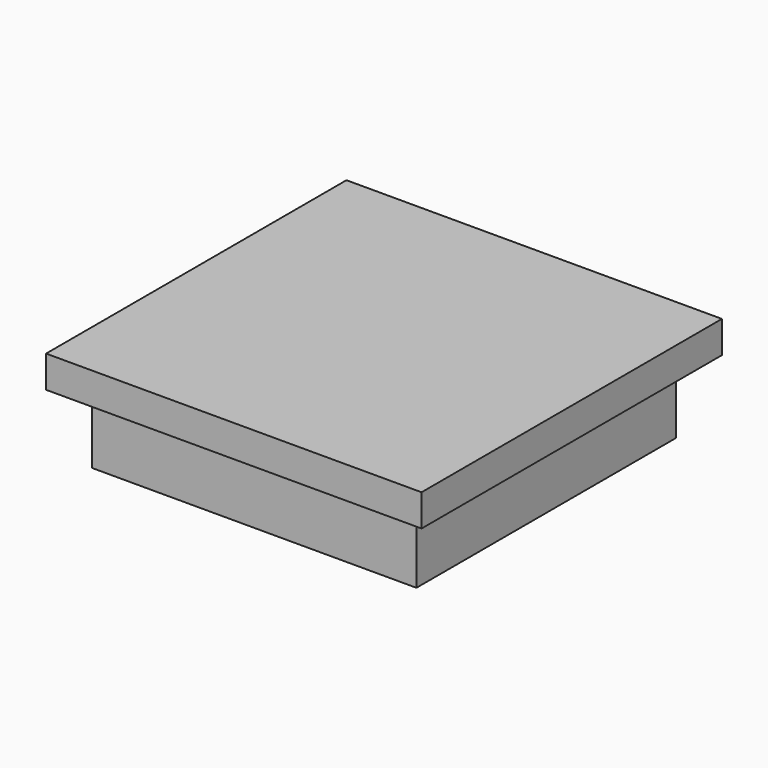
from build123d import *

# Parameters (mm, degrees)
F0_W     = 50.8
F0_H     = 50.8
F0_W_2   = 1
F0_H_2   = 8.95
F0_H_3   = 3
F1_DEPTH = 15
F2_DEPTH = 2
F3_R     = 5
F5_W     = 58.8
F5_H     = 58.8
F5_W_2   = 54.8
F5_H_2   = 54.8
F6_DEPTH = 5
F5_W_3   = 50.8
F5_H_3   = 50.8
F7_DEPTH = 2


with BuildPart() as f1:
    # F0 (on Top) → F1 (new body)
    with BuildSketch(Plane.XY):
        with Locations((-5.4668284297, -0.6229165018)):
            Rectangle(F0_W, F0_H)
        Polygon((-27.8668284297, 12.8270834982), (-27.8668284297, 21.7770834982), (-6.4668284297, 21.7770834982), (-5.4668284297, 21.7770834982), (-4.4668284297, 21.7770834982), (16.9331715703, 21.7770834982), (16.9331715703, 12.8270834982), (16.9331715703, 9.8270834982), (16.9331715703, 0.8770834982), (16.9331715703, -2.1229165018), (16.9331715703, -11.0729165018), (16.9331715703, -14.0729165018), (16.9331715703, -23.0229165018), (-4.4668284297, -23.0229165018), (-5.4668284297, -23.0229165018), (-6.4668284297, -23.0229165018), (-27.8668284297, -23.0229165018), (-27.8668284297, -14.0729165018), (-27.8668284297, -11.0729165018), (-27.8668284297, -2.1229165018), (-27.8668284297, 0.8770834982), (-27.8668284297, 9.8270834982), align=None, mode=Mode.SUBTRACT)
        with Locations((-5.9668284297, -6.5979165018)):
            Rectangle(F0_W_2, F0_H_2)
        with Locations((-4.9668284297, -6.5979165018)):
            Rectangle(F0_W_2, F0_H_2)
        with Locations((-5.9668284297, -12.5729165018)):
            Rectangle(F0_W_2, F0_H_3)
        with Locations((-4.9668284297, -12.5729165018)):
            Rectangle(F0_W_2, F0_H_3)
        with Locations((-5.9668284297, -18.5479165018)):
            Rectangle(F0_W_2, F0_H_2)
        with Locations((-4.9668284297, -18.5479165018)):
            Rectangle(F0_W_2, F0_H_2)
        with Locations((-5.9668284297, -0.6229165018)):
            Rectangle(F0_W_2, F0_H_3)
        with Locations((-4.9668284297, -0.6229165018)):
            Rectangle(F0_W_2, F0_H_3)
        with Locations((-5.9668284297, 5.3520834982)):
            Rectangle(F0_W_2, F0_H_2)
        with Locations((-4.9668284297, 5.3520834982)):
            Rectangle(F0_W_2, F0_H_2)
        with Locations((-5.9668284297, 17.3020834982)):
            Rectangle(F0_W_2, F0_H_2)
        with Locations((-4.9668284297, 17.3020834982)):
            Rectangle(F0_W_2, F0_H_2)
        with Locations((-5.9668284297, 11.3270834982)):
            Rectangle(F0_W_2, F0_H_3)
        with Locations((-4.9668284297, 11.3270834982)):
            Rectangle(F0_W_2, F0_H_3)
    extrude(amount=F1_DEPTH)

    # F0 (on Top) → F2 (join)
    with BuildSketch(Plane.XY):
        Polygon((-6.4668284297, 21.7770834982), (-27.8668284297, 21.7770834982), (-27.8668284297, 12.8270834982), (-27.8668284297, 9.8270834982), (-27.8668284297, 0.8770834982), (-27.8668284297, -2.1229165018), (-27.8668284297, -11.0729165018), (-27.8668284297, -14.0729165018), (-27.8668284297, -23.0229165018), (-6.4668284297, -23.0229165018), (-6.4668284297, -14.0729165018), (-6.4668284297, -11.0729165018), (-6.4668284297, -2.1229165018), (-6.4668284297, 0.8770834982), (-6.4668284297, 9.8270834982), (-6.4668284297, 12.8270834982), align=None)
        Polygon((16.9331715703, 21.7770834982), (-4.4668284297, 21.7770834982), (-4.4668284297, 12.8270834982), (-4.4668284297, 9.8270834982), (-4.4668284297, 0.8770834982), (-4.4668284297, -2.1229165018), (-4.4668284297, -11.0729165018), (-4.4668284297, -14.0729165018), (-4.4668284297, -23.0229165018), (16.9331715703, -23.0229165018), (16.9331715703, -14.0729165018), (16.9331715703, -11.0729165018), (16.9331715703, -2.1229165018), (16.9331715703, 0.8770834982), (16.9331715703, 9.8270834982), (16.9331715703, 12.8270834982), align=None)
    extrude(amount=F2_DEPTH)

    # F3
    f3_edges = [f1.edges().sort_by_distance(p)[0] for p in [
        (-27.866828, -23.022917, 8.5),
        (16.933172, -23.022917, 8.5),
        (-27.866828, 21.777083, 8.5),
        (16.933172, 21.777083, 8.5),
        (-4.466828, 21.777083, 8.5),
        (-6.466828, 21.777083, 8.5),
        (-6.466828, -23.022917, 8.5),
        (-4.466828, -23.022917, 8.5),
    ]]
    fillet(f3_edges, radius=F3_R)


with BuildPart() as f6:
    # F5 (on offset) → F6 (new body)
    with BuildSketch(Plane.XY.offset(16.1)):
        with Locations((-5.4668284297, -0.6229165018)):
            Rectangle(F5_W, F5_H)
        with Locations((-5.4668284297, -0.6229165018)):
            Rectangle(F5_W_2, F5_H_2, mode=Mode.SUBTRACT)
    extrude(amount=-F6_DEPTH)

    # F5 (on offset) → F7 (join)
    with BuildSketch(Plane.XY.offset(16.1)):
        with Locations((-5.4668284297, -0.6229165018)):
            Rectangle(F5_W_2, F5_H_2)
        with Locations((-5.4668284297, -0.6229165018)):
            Rectangle(F5_W_3, F5_H_3, mode=Mode.SUBTRACT)
        with Locations((-5.4668284297, -0.6229165018)):
            Rectangle(F5_W_3, F5_H_3)
    extrude(amount=-F7_DEPTH)


solid = Compound([f1.part, f6.part])
